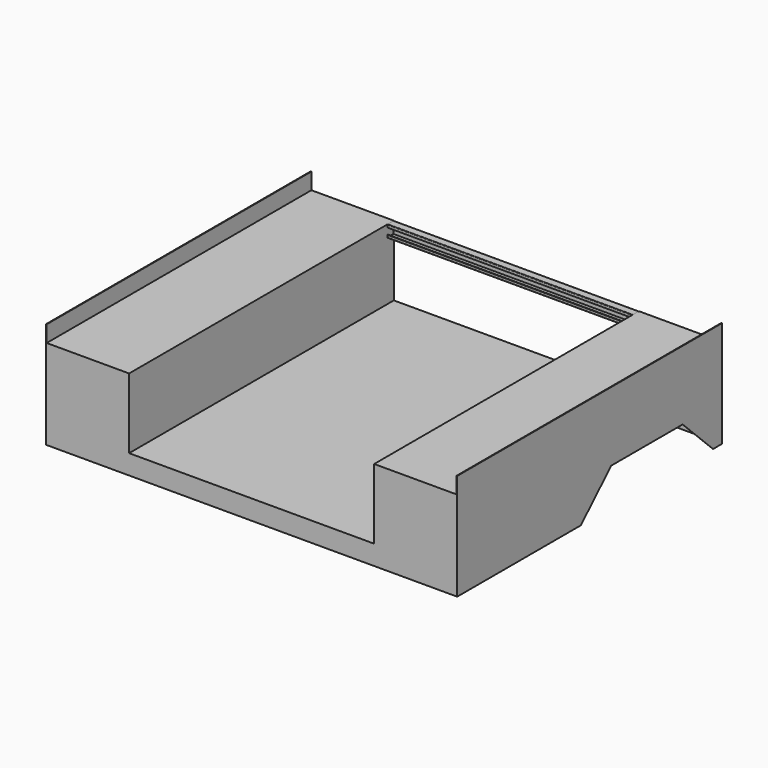
from build123d import *

# Parameters (mm, degrees)
F1_DEPTH      = 1650
F2_T          = 1.5
F2_T3_DEPTH   = 1653
F4_DEPTH      = 611
F4_DEPTH_BACK = 611
F8_DEPTH      = 1.5


# Not quite as in the source:
# - a shell that OpenCascade refuses in one call is made with other operations: the cavity is built on its own and cut out
# - the program builds the solid bodies; features that only make, move or delete a surface that nothing else refers to are left out


with BuildPart() as f1:
    # F0 (on Front) → F1 (new body)
    with BuildSketch(Plane.XZ):
        Polygon((-1025, 0), (1025, 0), (1025, 530), (1022, 530), (1022, 448), (611, 448), (611, 98), (-611, 98), (-611, 448), (-1022, 448), (-1022, 530), (-1025, 530), align=None)
    extrude(amount=F1_DEPTH)

    # F2: shell of thickness 1.5, made by hand


with BuildPart() as f2_core1:
    # F2_t2: copy of F1
    add(f1.part)

    # the walls: a layer under each face that stays
    f2_faces = [f2_core1.faces().sort_by_distance(p)[0] for p in [
        (1025, -825, 265),
        (1023.5, -825, 530),
        (1022, -825, 489),
        (816.5, -825, 448),
        (611, -825, 273),
        (0, -825, 98),
        (-611, -825, 273),
        (-816.5, -825, 448),
        (-1022, -825, 489),
        (-1023.5, -825, 530),
        (-1025, -825, 265),
        (-683.3333333333, 0, 88.3333333333),
        (-683.3333333333, -1650, 88.3333333333),
    ]]
    thicken(f2_faces, amount=-F2_T, mode=Mode.SUBTRACT)

    # F2_s4 → F2_t3 (cut)
    with BuildSketch(Plane.XZ.offset(-1.5)):
        Polygon((1021.985, 448.015), (1023.5, 448), (1023.5, 446.5), (1022, 446.5), align=None)
        Polygon((610.985, 98.015), (612.5, 98), (612.5, 96.5), (611, 96.5), align=None)
        Polygon((-610.985, 98.015), (-611, 96.5), (-612.5, 96.5), (-612.5, 98), align=None)
        Polygon((-1021.985, 448.015), (-1022, 446.5), (-1023.5, 446.5), (-1023.5, 448), align=None)
    extrude(amount=F2_T3_DEPTH, mode=Mode.SUBTRACT)


with BuildPart() as f1_1:
    add(f1.part)

    # what is left inside the walls is the cavity
    f2_cavity = [f2_core1.part.solids().sort_by_distance(p)[0] for p in [
        (0, -1099.5, 0.015),
    ]]
    add(f2_cavity, mode=Mode.SUBTRACT)

    # F7 (on face) → F8 (cut, through all)
    with BuildSketch(Plane.YZ.offset(1025)):
        Polygon((-879.4733192202, 0), (-55, 0), (-244.7366596101, 185), (-689.7366596101, 185), align=None)
    extrude(amount=-F8_DEPTH, mode=Mode.SUBTRACT)


with BuildPart() as f4:
    # F3 (on Right) → F4 (new body, two sides)
    with BuildSketch(Plane.YZ) as f4_sk:
        with BuildLine():
            Line((0, 391), (0, 445))
            ThreePointArc((0, 445), (-0.8786796564, 447.1213203436), (-3, 448))
            Line((-3, 448), (-37, 448))
            ThreePointArc((-37, 448), (-39.1213203436, 447.1213203436), (-40, 445))
            Line((-40, 445), (-40, 434))
            Line((-40, 434), (-37, 434))
            Line((-37, 434), (-37, 445))
            Line((-37, 445), (-3, 445))
            Line((-3, 445), (-3, 391))
            Line((-3, 391), (-37, 391))
            Line((-37, 391), (-37, 402))
            Line((-37, 402), (-40, 402))
            Line((-40, 402), (-40, 391))
            ThreePointArc((-40, 391), (-39.1213203436, 388.8786796564), (-37, 388))
            Line((-37, 388), (-3, 388))
            ThreePointArc((-3, 388), (-0.8786796564, 388.8786796564), (0, 391))
        make_face()
    extrude(amount=F4_DEPTH)
    extrude(f4_sk.sketch, amount=-F4_DEPTH_BACK)


solid = Compound([f1_1.part, f4.part])
